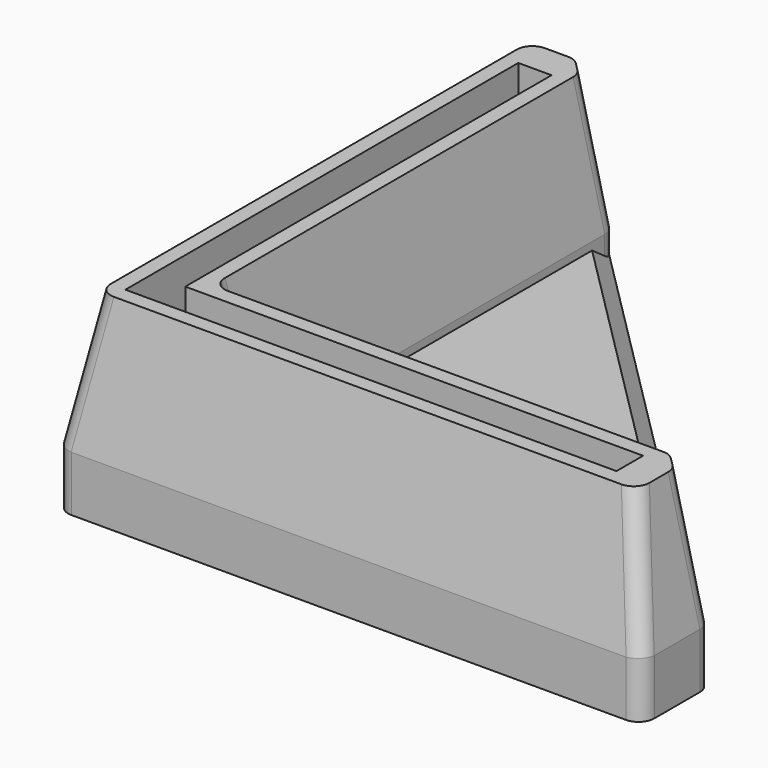
from build123d import *

# Parameters (mm, degrees)
F1_DEPTH  = 3
F3_DEPTH  = 9
F5_DEPTH  = 9
F7_DEPTH  = 25
F9_DEPTH  = 25
F10_SIZE2 = 8.5069227294
F10_SIZE  = 1.5
F11_SIZE  = 1
F12_F1_R  = 1
F12_F2_R  = 1
F12_F3_R  = 1
F12_F4_R  = 1
F12_F5_R  = 1
F12_F6_R  = 1
F12_F7_R  = 1
F12_F8_R  = 1
F12_F9_R  = 1
F12_F10_R = 1
F12_F11_R = 1
F12_F12_R = 1
F12_F13_R = 1
F12_F14_R = 1
F12_F15_R = 1


with BuildPart() as f1:
    # F0 (on Top) → F1 (new body)
    with BuildSketch(Plane.XY):
        Polygon((0, 0), (-42, 42), (-42, 0), align=None)
    extrude(amount=F1_DEPTH)

    # F2 (on face) → F3 (join)
    with BuildSketch(Plane.XY.offset(3)):
        Polygon((-42, 37), (-42, 0), (-5, 0), (-5, 5), (-7, 7), (-35, 7), (-35, 35), (-37, 37), align=None)
    extrude(amount=F3_DEPTH)

    # F4 (on face) → F5 (cut)
    with BuildSketch(Plane.XY.offset(12)):
        Polygon((-39.55, 33.45), (-39.55, 2.45), (-8.55, 2.45), (-8.55, 4.55), (-37.45, 4.55), (-37.45, 33.45), align=None)
    extrude(amount=-F5_DEPTH, mode=Mode.SUBTRACT)

    # F6 (on face) → F7 (cut)
    with BuildSketch(Plane.XY.offset(3)):
        Polygon((-5, 5), (-5, 0), (0, 0), align=None)
    extrude(amount=-F7_DEPTH, mode=Mode.SUBTRACT)

    # F8 (on face) → F9 (cut)
    with BuildSketch(Plane.XY.offset(3)):
        Polygon((-42, 42), (-42, 37), (-37, 37), align=None)
    extrude(amount=-F9_DEPTH, mode=Mode.SUBTRACT)

    # F10
    f10_edges = [f1.edges().sort_by_distance(p)[0] for p in [
        (-23.5, 0, 12),
        (-5, 2.5, 12),
        (-6, 6, 12),
        (-21, 7, 12),
        (-35, 21, 12),
        (-36, 36, 12),
        (-39.5, 37, 12),
        (-42, 18.5, 12),
    ]]
    f10_side = f1.faces().sort_by_distance((-41.476741, 18.5, 12))[0]
    chamfer(f10_edges, length=F10_SIZE, length2=F10_SIZE2, reference=f10_side)

    # F11
    f11_edges = [f1.edges().sort_by_distance(p)[0] for p in [
        (-21, 21, 3),
    ]]
    chamfer(f11_edges, length=F11_SIZE)

    # F12: fillet of radius 1 on 17 edges, made by hand

    # F12_f1
    f12_f1_edges = [f1.edges().sort_by_distance(p)[0] for p in [
        (-7, 7, 2.5),
        (-7, 7, 3.2465386353),
    ]]
    fillet(f12_f1_edges, radius=F12_F1_R)

    # F12_f2
    f12_f2_edges = [f1.edges().sort_by_distance(p)[0] for p in [
        (-35, 35, 2.5),
        (-35, 35, 3.2465386353),
    ]]
    fillet(f12_f2_edges, radius=F12_F2_R)

    # F12_f3
    f12_f3_edges = [f1.edges().sort_by_distance(p)[0] for p in [
        (-5, 5, 1.7465386353),
    ]]
    fillet(f12_f3_edges, radius=F12_F3_R)

    # F12_f4
    f12_f4_edges = [f1.edges().sort_by_distance(p)[0] for p in [
        (-37, 37, 1.7465386353),
    ]]
    fillet(f12_f4_edges, radius=F12_F4_R)

    # F12_f5
    f12_f5_edges = [f1.edges().sort_by_distance(p)[0] for p in [
        (-5.7880602337, 4.6735747632, 7.962388947),
    ]]
    fillet(f12_f5_edges, radius=F12_F5_R)

    # F12_f6
    f12_f6_edges = [f1.edges().sort_by_distance(p)[0] for p in [
        (-7.3264252368, 6.2119397663, 7.962388947),
    ]]
    fillet(f12_f6_edges, radius=F12_F6_R)

    # F12_f7
    f12_f7_edges = [f1.edges().sort_by_distance(p)[0] for p in [
        (-5, 0, 1.7465386353),
    ]]
    fillet(f12_f7_edges, radius=F12_F7_R)

    # F12_f8
    f12_f8_edges = [f1.edges().sort_by_distance(p)[0] for p in [
        (-35.7880602337, 34.6735747632, 7.962388947),
    ]]
    fillet(f12_f8_edges, radius=F12_F8_R)

    # F12_f9
    f12_f9_edges = [f1.edges().sort_by_distance(p)[0] for p in [
        (-37.3264252368, 36.2119397663, 7.962388947),
    ]]
    fillet(f12_f9_edges, radius=F12_F9_R)

    # F12_f10
    f12_f10_edges = [f1.edges().sort_by_distance(p)[0] for p in [
        (-42, 37, 1.7465386353),
    ]]
    fillet(f12_f10_edges, radius=F12_F10_R)

    # F12_f11
    f12_f11_edges = [f1.edges().sort_by_distance(p)[0] for p in [
        (-35.75, 6.25, 7.7465386353),
    ]]
    fillet(f12_f11_edges, radius=F12_F11_R)

    # F12_f12
    f12_f12_edges = [f1.edges().sort_by_distance(p)[0] for p in [
        (-5.8964466094, 0.8964466094, 8.5770786288),
    ]]
    fillet(f12_f12_edges, radius=F12_F12_R)

    # F12_f13
    f12_f13_edges = [f1.edges().sort_by_distance(p)[0] for p in [
        (-42, 0, 1.7465386353),
    ]]
    fillet(f12_f13_edges, radius=F12_F13_R)

    # F12_f14
    f12_f14_edges = [f1.edges().sort_by_distance(p)[0] for p in [
        (-41.1035533906, 36.1035533906, 8.5770786288),
    ]]
    fillet(f12_f14_edges, radius=F12_F14_R)

    # F12_f15
    f12_f15_edges = [f1.edges().sort_by_distance(p)[0] for p in [
        (-41.1035533906, 0.8964466094, 8.5770786288),
    ]]
    fillet(f12_f15_edges, radius=F12_F15_R)


solid = f1.part
